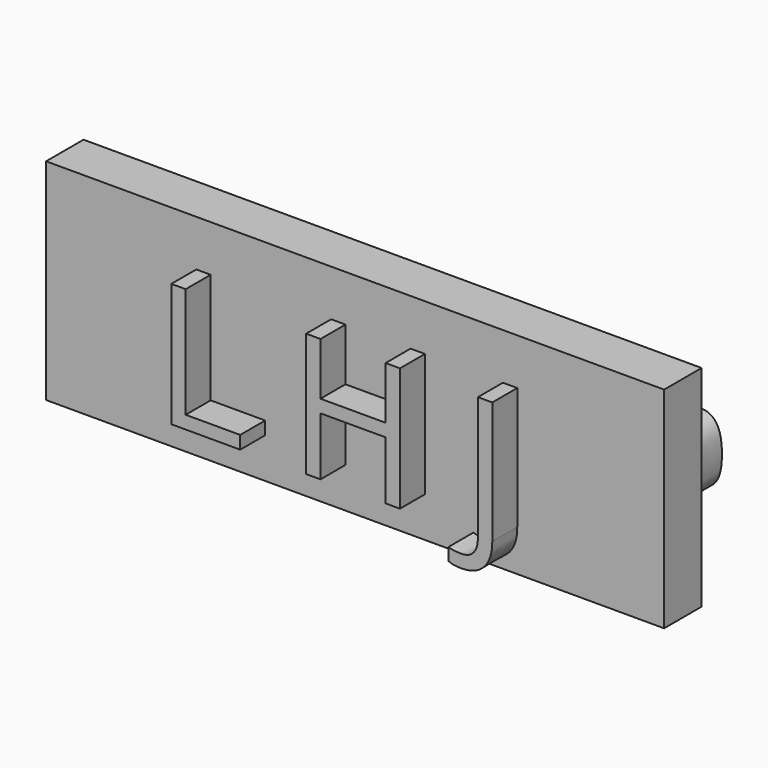
from build123d import *

# Parameters (mm, degrees)
F0_W         = 100.5655601621
F0_H         = 34.1978222132
F1_DEPTH     = 7.62
F2_TEXT_SIZE = 28.165321823
F3_DEPTH     = 5.08
F4_TEXT_SIZE = 15.0034869933
F5_DEPTH     = 5.08


# Not quite as in the source:
# - Text() gives the source's letters only with a copy of the font that has no kerning and outlines rounded to 1/6400 em; it was checked with that copy


with BuildPart() as f1:
    # F0 (on Front) → F1 (new body)
    with BuildSketch(Plane.XZ):
        with Locations((50.282780081, 17.0989111066)):
            Rectangle(F0_W, F0_H)
    extrude(amount=F1_DEPTH)

    # F2 (on face) → F3 (join)
    with BuildSketch(Plane.XZ.offset(7.62)):
        with Locations((21.6770414263, 6.5445983782)):
            Text('L H J', F2_TEXT_SIZE, font='Open Sans', text_align=(TextAlign.LEFT, TextAlign.BOTTOM))
    extrude(amount=F3_DEPTH)

    # F4 (on face) → F5 (join)
    with BuildSketch(Plane(origin=(0, 0, 0), x_dir=(-1, 0, 0), z_dir=(0, 1, 0))):
        with Locations((-100.5655601621, 14.1322263095)):
            Text('010262671951', F4_TEXT_SIZE, font='Open Sans', text_align=(TextAlign.LEFT, TextAlign.BOTTOM))
    extrude(amount=F5_DEPTH)


solid = f1.part
